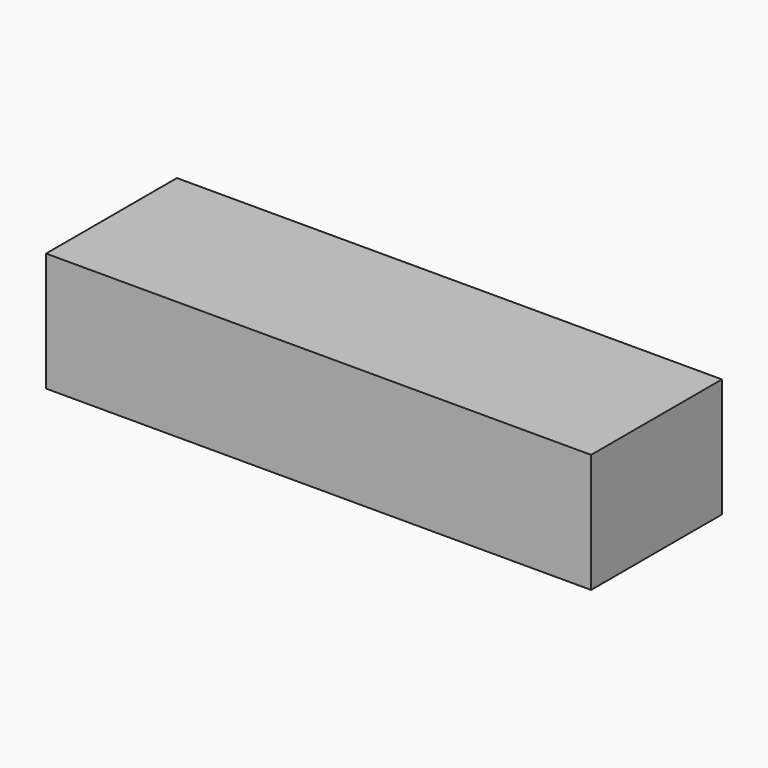
from build123d import *

# Parameters (mm, degrees)
F0_W     = 110
F0_H     = 33
F1_DEPTH = 24
F2_W     = 20
F2_H     = 15
F2_R     = 1.5
F2_W_2   = 3.9
F2_H_2   = 3.9
F3_DEPTH = 1.5
F4_DEPTH = 2.35


with BuildPart() as f1:
    # F0 (on Top) → F1 (new body)
    with BuildSketch(Plane.XY):
        Rectangle(F0_W, F0_H)
    extrude(amount=F1_DEPTH)


with BuildPart() as f3:
    # F2 (on Top) → F3 (new body)
    with BuildSketch(Plane.XY):
        Rectangle(F2_W, F2_H)
        with Locations((-7.5, 5)):
            Circle(F2_R, mode=Mode.SUBTRACT)
        Rectangle(F2_W_2, F2_H_2, mode=Mode.SUBTRACT)
        with Locations((7.5, 5)):
            Circle(F2_R, mode=Mode.SUBTRACT)
    extrude(amount=F3_DEPTH)

    # F2 (on Top) → F4 (join)
    with BuildSketch(Plane.XY):
        Rectangle(F2_W_2, F2_H_2)
    extrude(amount=F4_DEPTH)


solid = Compound([f1.part, f3.part])
